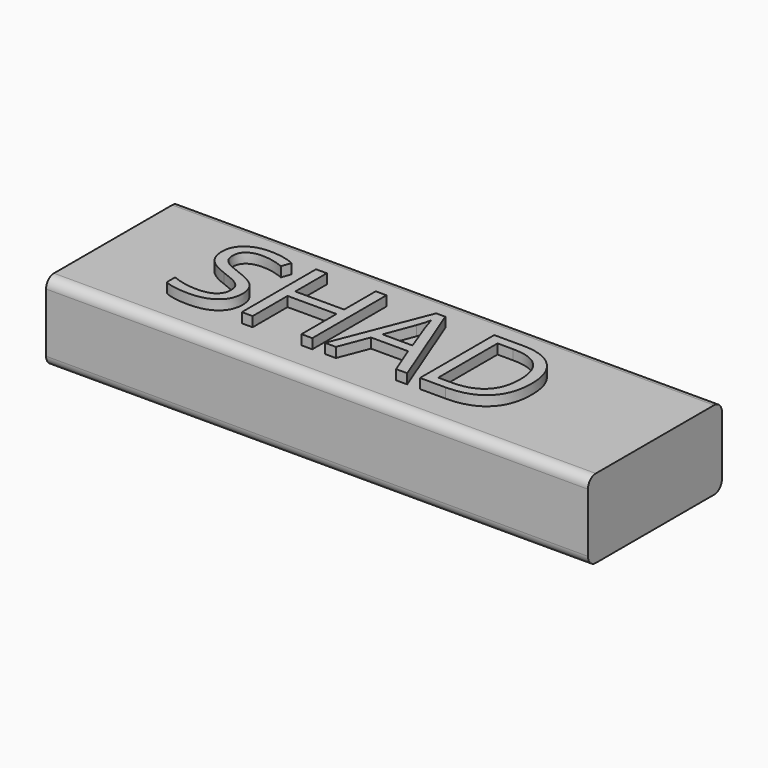
from build123d import *

# Parameters (mm, degrees)
F1_DEPTH     = 55
F2_W         = 12.4
F2_H         = 5
F3_DEPTH     = 14
F4_ANGLE     = 90
F5_TEXT_SIZE = 13.1940313925
F6_DEPTH     = 1


# Not quite as in the source:
# - Text() gives the source's letters only with a copy of the font that has no kerning and outlines rounded to 1/6400 em; it was checked with that copy


with BuildPart() as f1:
    # F0 (on Front) → F1 (new body)
    with BuildSketch(Plane.XZ):
        with BuildLine():
            Line((7.5, 4), (-7.5, 4))
            ThreePointArc((-7.5, 4), (-8.2071067812, 3.7071067812), (-8.5, 3))
            Line((-8.5, 3), (-8.5, -3))
            ThreePointArc((-8.5, -3), (-8.2071067812, -3.7071067812), (-7.5, -4))
            Line((-7.5, -4), (7.5, -4))
            ThreePointArc((7.5, -4), (8.2071067812, -3.7071067812), (8.5, -3))
            Line((8.5, -3), (8.5, 3))
            ThreePointArc((8.5, 3), (8.2071067812, 3.7071067812), (7.5, 4))
        make_face()
    extrude(amount=F1_DEPTH)

    # F2 (on face) → F3 (cut)
    with BuildSketch(Plane.XZ.offset(55)):
        Rectangle(F2_W, F2_H)
    extrude(amount=-F3_DEPTH, mode=Mode.SUBTRACT)


with BuildPart() as f1_1:
    # F4: moved
    add(f1.part.rotate(Axis((8.5, -55, 0), (0, 0, -1)), F4_ANGLE))

    # F5 (on face) → F6 (join)
    with BuildSketch(Plane.XY.offset(4)):
        with Locations((16.9540345669, -51.4043234289)):
            Text('SHAD', F5_TEXT_SIZE, font='Open Sans', text_align=(TextAlign.LEFT, TextAlign.BOTTOM))
    extrude(amount=F6_DEPTH)


solid = f1_1.part
